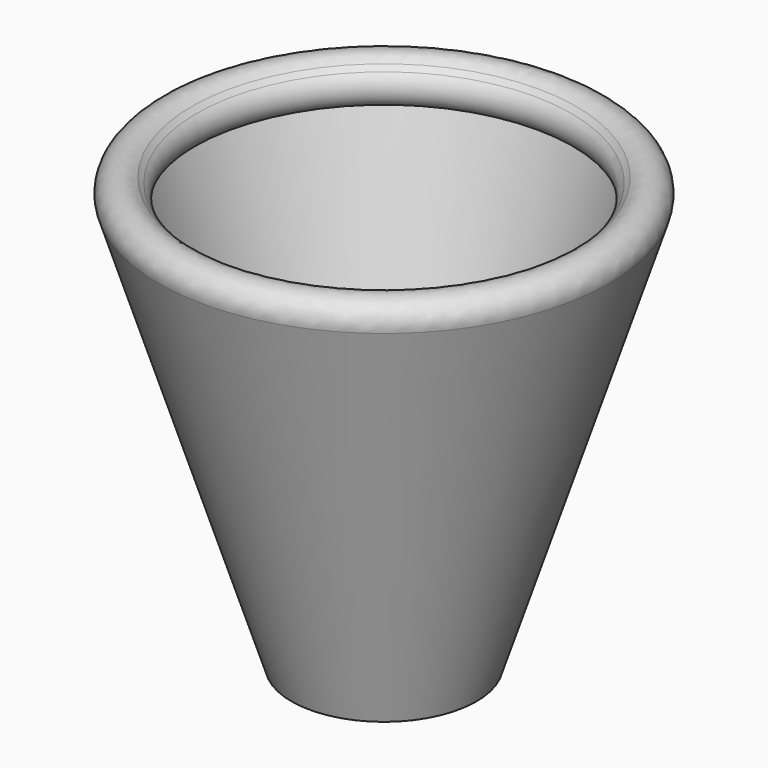
from build123d import *

# Parameters (mm, degrees)
F2_R = 5.08


# Not quite as in the source:
# - a fillet or chamfer that OpenCascade refuses, or shapes differently, is made with other operations: its cross-section is extruded or revolved along the edge and cut away or added


with BuildPart() as f1:
    # F0 (on Right) → F1 (revolve)
    with BuildSketch(Plane.YZ):
        Polygon((31.2051475048, 40.8137366176), (0, 38.317322731), (0, -51.5535026789), (23.7159132957, -51.5535026789), (64.1577839851, 73.7663730979), align=None)
    revolve(axis=Axis((0, 0, -6.6180899739), (0, 0, -1)))

    # F2
    f2_edges = [f1.edges().sort_by_distance(p)[0] for p in [
        (0, -64.157784, 73.766373),
    ]]
    fillet(f2_edges, radius=F2_R)

    # F3 (on Front) → F4 (revolve, cut)
    with BuildSketch(Plane.XZ):
        Polygon((48.9296764135, 49.8008169234), (0, 49.8008169234), (0, -34.0786203742), (22.218067199, -34.0786203742), align=None)
    revolve(axis=Axis((0, 0, 7.8610982746), (0, 0, -1)), mode=Mode.SUBTRACT)

    # F5: fillet of radius 5.08 on 1 edges, made by hand

    # F5_s1 → F5_t2 (revolve, cut)
    with BuildSketch(Plane.YZ):
        with BuildLine():
            ThreePointArc((48.0680960352, 57.6766851479), (46.6103251908, 53.5321519556), (48.9296764135, 49.8008169234))
            Line((48.9296764135, 49.8008169234), (48.8750659721, 49.7151416079))
            ThreePointArc((48.8750659721, 49.7151416079), (44.5609521121, 49.6992169234), (40.1922278106, 49.6992169234))
            Line((40.1922278106, 49.6992169234), (40.1203857617, 49.8726589723))
            Line((40.1203857617, 49.8726589723), (47.9962539862, 57.7485271969))
            Line((47.9962539862, 57.7485271969), (48.0680960352, 57.6766851479))
        make_face()
    revolve(axis=Axis((0, 0, 49.8008169234), (0, 0, -1)), mode=Mode.SUBTRACT)


solid = f1.part
